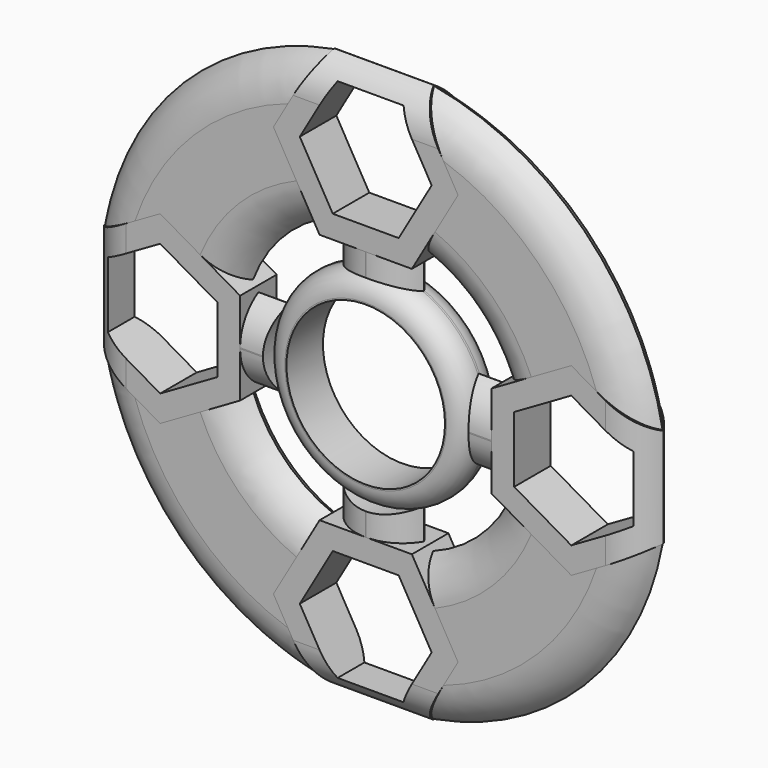
from build123d import *

# Parameters (mm, degrees)
F0_R          = 14.2875
F0_R_2        = 11.0236
F2_DEPTH      = 6.35
F3_T2_ANGLE   = 116.8949304421
F3_T4_ANGLE   = 116.8949304421
F3_2_T2_ANGLE = 116.8949304421
F3_2_T4_ANGLE = 116.8949304421
F3_3_T2_ANGLE = 116.8949304421
F3_3_T4_ANGLE = 116.8949304421
F3_4_T2_ANGLE = 116.8949304421
F3_4_T4_ANGLE = 116.8949304421
F3_5_T1_DEPTH = 44.5816097327
F3_6_T1_DEPTH = 44.5816097327
F3_7_T1_DEPTH = 44.5816097327
F3_8_T1_DEPTH = 44.5816097327
F4_T1_DEPTH   = 36.4465255301
F4_2_T1_DEPTH = 36.4465255301
F4_3_T1_DEPTH = 36.4465255301
F4_4_T1_DEPTH = 36.4465255301
F5_T2_ANGLE   = 147.4481035584
F5_T4_ANGLE   = 147.4481035584
F5_2_T2_ANGLE = 147.4481035584
F5_2_T4_ANGLE = 147.4481035584
F5_3_T2_ANGLE = 147.4481035584
F5_3_T4_ANGLE = 147.4481035584
F5_4_T2_ANGLE = 147.4481035584
F5_4_T4_ANGLE = 147.4481035584
F6_R          = 3.048


# Not quite as in the source:
# - a fillet or chamfer that OpenCascade refuses, or shapes differently, is made with other operations: its cross-section is extruded or revolved along the edge and cut away or added


with BuildPart() as f2:
    # F0 (on Front) → F2 (new body)
    with BuildSketch(Plane.XZ):
        Circle(F0_R)
        Circle(F0_R_2, mode=Mode.SUBTRACT)
    extrude(amount=F2_DEPTH)

    # F6
    f6_edges = [f2.edges().sort_by_distance(p)[0] for p in [
        (-14.2875, 0, 0),
        (-14.2875, -6.35, 0),
    ]]
    fillet(f6_edges, radius=F6_R)


with BuildPart() as f2b:
    # F0 (on Front) → F2, piece 2 (new body)
    with BuildSketch(Plane.XZ):
        Polygon((-6.4158048664, 17.4625), (6.4158048664, 17.4625), (12.8316097327, 28.575), (6.4158048664, 39.6875), (-6.4158048664, 39.6875), (-12.8316097327, 28.575), align=None)
        Polygon((9.1654355234, 28.575), (4.5827177617, 20.6375), (-4.5827177617, 20.6375), (-9.1654355234, 28.575), (-4.5827177617, 36.5125), (4.5827177617, 36.5125), align=None, mode=Mode.SUBTRACT)
    extrude(amount=F2_DEPTH)

    # F3#5: fillet of radius 6.35 on 2 edges, made by hand

    # F3_5_s2 → F3_5_t1 (cut)
    with BuildSketch(Plane.YZ.offset(-22.2908048664)):
        with BuildLine():
            ThreePointArc((0, 39.6875), (-4.4901280605, 37.8276280605), (-6.35, 33.3375))
            Line((-6.35, 33.3375), (-6.35, 39.6875))
            Line((-6.35, 39.6875), (0, 39.6875))
        make_face()
        with BuildLine():
            ThreePointArc((-6.35, 39.6875), (-1.8598719395, 37.8276280605), (0, 33.3375))
            Line((0, 33.3375), (0, 39.6875))
            Line((0, 39.6875), (-6.35, 39.6875))
        make_face()
    extrude(amount=F3_5_T1_DEPTH, mode=Mode.SUBTRACT)


with BuildPart() as f2c:
    # F0 (on Front) → F2, piece 3 (new body)
    with BuildSketch(Plane.XZ):
        Polygon((-17.4625, 6.4158048664), (-28.575, 12.8316097327), (-39.6875, 6.4158048664), (-39.6875, -6.4158048664), (-28.575, -12.8316097327), (-17.4625, -6.4158048664), align=None)
        Polygon((-28.575, 9.1654355234), (-20.6375, 4.5827177617), (-20.6375, -4.5827177617), (-28.575, -9.1654355234), (-36.5125, -4.5827177617), (-36.5125, 4.5827177617), align=None, mode=Mode.SUBTRACT)
    extrude(amount=F2_DEPTH)

    # F3#6: fillet of radius 6.35 on 2 edges, made by hand

    # F3_6_s2 → F3_6_t1 (cut)
    with BuildSketch(Plane.XY.offset(-22.2908048664)):
        with BuildLine():
            ThreePointArc((-39.6875, 0), (-37.8276280605, -4.4901280605), (-33.3375, -6.35))
            Line((-33.3375, -6.35), (-39.6875, -6.35))
            Line((-39.6875, -6.35), (-39.6875, 0))
        make_face()
        with BuildLine():
            ThreePointArc((-39.6875, -6.35), (-37.8276280605, -1.8598719395), (-33.3375, 0))
            Line((-33.3375, 0), (-39.6875, 0))
            Line((-39.6875, 0), (-39.6875, -6.35))
        make_face()
    extrude(amount=F3_6_T1_DEPTH, mode=Mode.SUBTRACT)


with BuildPart() as f2d:
    # F0 (on Front) → F2, piece 4 (new body)
    with BuildSketch(Plane.XZ):
        Polygon((-6.4158048664, -17.4625), (-12.8316097327, -28.575), (-6.4158048664, -39.6875), (6.4158048664, -39.6875), (12.8316097327, -28.575), (6.4158048664, -17.4625), align=None)
        Polygon((-9.1654355234, -28.575), (-4.5827177617, -20.6375), (4.5827177617, -20.6375), (9.1654355234, -28.575), (4.5827177617, -36.5125), (-4.5827177617, -36.5125), align=None, mode=Mode.SUBTRACT)
    extrude(amount=F2_DEPTH)

    # F3#8: fillet of radius 6.35 on 2 edges, made by hand

    # F3_8_s2 → F3_8_t1 (cut)
    with BuildSketch(Plane.YZ.offset(-22.2908048664)):
        with BuildLine():
            ThreePointArc((0, -39.6875), (-4.4901280605, -37.8276280605), (-6.35, -33.3375))
            Line((-6.35, -33.3375), (-6.35, -39.6875))
            Line((-6.35, -39.6875), (0, -39.6875))
        make_face()
        with BuildLine():
            ThreePointArc((-6.35, -39.6875), (-1.8598719395, -37.8276280605), (0, -33.3375))
            Line((0, -33.3375), (0, -39.6875))
            Line((0, -39.6875), (-6.35, -39.6875))
        make_face()
    extrude(amount=F3_8_T1_DEPTH, mode=Mode.SUBTRACT)


with BuildPart() as f2e:
    # F0 (on Front) → F2, piece 5 (new body)
    with BuildSketch(Plane.XZ):
        Polygon((17.4625, -6.4158048664), (28.575, -12.8316097327), (39.6875, -6.4158048664), (39.6875, 6.4158048664), (28.575, 12.8316097327), (17.4625, 6.4158048664), align=None)
        Polygon((28.575, -9.1654355234), (20.6375, -4.5827177617), (20.6375, 4.5827177617), (28.575, 9.1654355234), (36.5125, 4.5827177617), (36.5125, -4.5827177617), align=None, mode=Mode.SUBTRACT)
    extrude(amount=F2_DEPTH)

    # F3#7: fillet of radius 6.35 on 2 edges, made by hand

    # F3_7_s2 → F3_7_t1 (cut)
    with BuildSketch(Plane.XY.offset(-22.2908048664)):
        with BuildLine():
            ThreePointArc((39.6875, 0), (37.8276280605, -4.4901280605), (33.3375, -6.35))
            Line((33.3375, -6.35), (39.6875, -6.35))
            Line((39.6875, -6.35), (39.6875, 0))
        make_face()
        with BuildLine():
            ThreePointArc((39.6875, -6.35), (37.8276280605, -1.8598719395), (33.3375, 0))
            Line((33.3375, 0), (39.6875, 0))
            Line((39.6875, 0), (39.6875, -6.35))
        make_face()
    extrude(amount=F3_7_T1_DEPTH, mode=Mode.SUBTRACT)


with BuildPart() as f2f:
    # F1 (on Front) → F2, piece 6 (new body)
    with BuildSketch(Plane.XZ):
        with BuildLine():
            ThreePointArc((-6.4158048664, 39.6875), (-28.4276292393, 28.4276292393), (-39.6875, 6.4158048664))
            Line((-39.6875, 6.4158048664), (-34.1312501453, 9.6237072156))
            Line((-34.1312501453, 9.6237072156), (-28.575, 12.8316097327))
            Line((-28.575, 12.8316097327), (-23.0187499915, 9.6237072946))
            Line((-23.0187499915, 9.6237072946), (-17.4625, 6.4158048664))
            ThreePointArc((-17.4625, 6.4158048664), (-13.1548747302, 13.1548747302), (-6.4158048664, 17.4625))
            Line((-6.4158048664, 17.4625), (-9.6237073033, 23.0187500066))
            Line((-9.6237073033, 23.0187500066), (-12.8316097327, 28.575))
            Line((-12.8316097327, 28.575), (-9.6237073033, 34.1312499934))
            Line((-9.6237073033, 34.1312499934), (-6.4158048664, 39.6875))
        make_face()
    extrude(amount=F2_DEPTH)

    # F3#4: fillet of radius 6.35 on 2 edges, made by hand

    # F3_4_s1 → F3_4_t2 (revolve, cut)
    with BuildSketch(Plane(origin=(0, 0, 0), x_dir=(0, 1, 0), z_dir=(0.9725835588, 0, -0.2325536951))):
        with BuildLine():
            ThreePointArc((0, 40.2027388163), (-4.4901280605, 38.3428668769), (-6.35, 33.8527388163))
            Line((-6.35, 33.8527388163), (-6.35, 40.2027388163))
            Line((-6.35, 40.2027388163), (0, 40.2027388163))
        make_face()
    revolve(axis=Axis((0, -6.35, 0), (0, -1, 0)), revolution_arc=F3_4_T2_ANGLE, mode=Mode.SUBTRACT)

    # F3_4_s3 → F3_4_t4 (revolve, cut)
    with BuildSketch(Plane(origin=(0, 0, 0), x_dir=(0, 1, 0), z_dir=(0.9725835588, 0, -0.2325536951))):
        with BuildLine():
            ThreePointArc((0, 33.8527388163), (-1.8598719395, 38.3428668769), (-6.35, 40.2027388163))
            Line((-6.35, 40.2027388163), (0, 40.2027388163))
            Line((0, 40.2027388163), (0, 33.8527388163))
        make_face()
    revolve(axis=Axis((0, 0, 0), (0, -1, 0)), revolution_arc=F3_4_T4_ANGLE, mode=Mode.SUBTRACT)

    # F5: fillet of radius 6.35 on 2 edges, made by hand

    # F5_s1 → F5_t2 (revolve, cut)
    with BuildSketch(Plane(origin=(0, 0, 0), x_dir=(0, 1, 0), z_dir=(0.4805916659, 0, -0.8769444969))):
        with BuildLine():
            ThreePointArc((-6.35, -24.9538022547), (-4.4901280605, -20.4636741942), (0, -18.6038022547))
            Line((0, -18.6038022547), (-6.35, -18.6038022547))
            Line((-6.35, -18.6038022547), (-6.35, -24.9538022547))
        make_face()
    revolve(axis=Axis((0, -6.35, 0), (0, 1, 0)), revolution_arc=F5_T2_ANGLE, mode=Mode.SUBTRACT)

    # F5_s3 → F5_t4 (revolve, cut)
    with BuildSketch(Plane(origin=(0, 0, 0), x_dir=(0, 1, 0), z_dir=(0.4805916659, 0, -0.8769444969))):
        with BuildLine():
            ThreePointArc((0, -24.9538022547), (-1.8598719395, -20.4636741942), (-6.35, -18.6038022547))
            Line((-6.35, -18.6038022547), (0, -18.6038022547))
            Line((0, -18.6038022547), (0, -24.9538022547))
        make_face()
    revolve(axis=Axis((0, 0, 0), (0, 1, 0)), revolution_arc=F5_T4_ANGLE, mode=Mode.SUBTRACT)


with BuildPart() as f2g:
    # F1 (on Front) → F2, piece 7 (new body)
    with BuildSketch(Plane.XZ):
        with BuildLine():
            Line((34.1312500085, 9.6237072946), (39.6875, 6.4158048664))
            ThreePointArc((39.6875, 6.4158048664), (28.4276292393, 28.4276292393), (6.4158048664, 39.6875))
            Line((6.4158048664, 39.6875), (9.6237073207, 34.1312499633))
            Line((9.6237073207, 34.1312499633), (12.8316097327, 28.575))
            Line((12.8316097327, 28.575), (9.6237072806, 23.0187499671))
            Line((9.6237072806, 23.0187499671), (6.4158048664, 17.4625))
            ThreePointArc((6.4158048664, 17.4625), (13.1548747302, 13.1548747302), (17.4625, 6.4158048664))
            Line((17.4625, 6.4158048664), (23.0187500159, 9.6237073087))
            Line((23.0187500159, 9.6237073087), (28.575, 12.8316097327))
            Line((28.575, 12.8316097327), (34.1312500085, 9.6237072946))
        make_face()
    extrude(amount=F2_DEPTH)

    # F3: fillet of radius 6.35 on 2 edges, made by hand

    # F3_s1 → F3_t2 (revolve, cut)
    with BuildSketch(Plane(origin=(0, 0, 0), x_dir=(0, 1, 0), z_dir=(-0.2325536951, 0, -0.9725835588))):
        with BuildLine():
            ThreePointArc((0, 40.2027388163), (-4.4901280605, 38.3428668769), (-6.35, 33.8527388163))
            Line((-6.35, 33.8527388163), (-6.35, 40.2027388163))
            Line((-6.35, 40.2027388163), (0, 40.2027388163))
        make_face()
    revolve(axis=Axis((0, -6.35, 0), (0, -1, 0)), revolution_arc=F3_T2_ANGLE, mode=Mode.SUBTRACT)

    # F3_s3 → F3_t4 (revolve, cut)
    with BuildSketch(Plane(origin=(0, 0, 0), x_dir=(0, 1, 0), z_dir=(-0.2325536951, 0, -0.9725835588))):
        with BuildLine():
            ThreePointArc((0, 33.8527388163), (-1.8598719395, 38.3428668769), (-6.35, 40.2027388163))
            Line((-6.35, 40.2027388163), (0, 40.2027388163))
            Line((0, 40.2027388163), (0, 33.8527388163))
        make_face()
    revolve(axis=Axis((0, 0, 0), (0, -1, 0)), revolution_arc=F3_T4_ANGLE, mode=Mode.SUBTRACT)

    # F5#4: fillet of radius 6.35 on 2 edges, made by hand

    # F5_4_s1 → F5_4_t2 (revolve, cut)
    with BuildSketch(Plane(origin=(0, 0, 0), x_dir=(0, 1, 0), z_dir=(-0.8769444969, 0, -0.4805916659))):
        with BuildLine():
            ThreePointArc((-6.35, -24.9538022547), (-4.4901280605, -20.4636741942), (0, -18.6038022547))
            Line((0, -18.6038022547), (-6.35, -18.6038022547))
            Line((-6.35, -18.6038022547), (-6.35, -24.9538022547))
        make_face()
    revolve(axis=Axis((0, -6.35, 0), (0, 1, 0)), revolution_arc=F5_4_T2_ANGLE, mode=Mode.SUBTRACT)

    # F5_4_s3 → F5_4_t4 (revolve, cut)
    with BuildSketch(Plane(origin=(0, 0, 0), x_dir=(0, 1, 0), z_dir=(-0.8769444969, 0, -0.4805916659))):
        with BuildLine():
            ThreePointArc((0, -24.9538022547), (-1.8598719395, -20.4636741942), (-6.35, -18.6038022547))
            Line((-6.35, -18.6038022547), (0, -18.6038022547))
            Line((0, -18.6038022547), (0, -24.9538022547))
        make_face()
    revolve(axis=Axis((0, 0, 0), (0, 1, 0)), revolution_arc=F5_4_T4_ANGLE, mode=Mode.SUBTRACT)


with BuildPart() as f2h:
    # F1 (on Front) → F2, piece 8 (new body)
    with BuildSketch(Plane.XZ):
        with BuildLine():
            Line((9.6237072946, -23.0187499915), (12.8316097327, -28.575))
            Line((12.8316097327, -28.575), (9.6237072946, -34.1312500085))
            Line((9.6237072946, -34.1312500085), (6.4158048664, -39.6875))
            ThreePointArc((6.4158048664, -39.6875), (28.4276292393, -28.4276292393), (39.6875, -6.4158048664))
            Line((39.6875, -6.4158048664), (34.1312500668, -9.623707261))
            Line((34.1312500668, -9.623707261), (28.575, -12.8316097327))
            Line((28.575, -12.8316097327), (23.0187499915, -9.6237072946))
            Line((23.0187499915, -9.6237072946), (17.4625, -6.4158048664))
            ThreePointArc((17.4625, -6.4158048664), (13.1548747302, -13.1548747302), (6.4158048664, -17.4625))
            Line((6.4158048664, -17.4625), (9.6237072946, -23.0187499915))
        make_face()
    extrude(amount=F2_DEPTH)

    # F3#2: fillet of radius 6.35 on 2 edges, made by hand

    # F3_2_s1 → F3_2_t2 (revolve, cut)
    with BuildSketch(Plane(origin=(0, 0, 0), x_dir=(0, 1, 0), z_dir=(-0.9725835588, 0, 0.2325536951))):
        with BuildLine():
            ThreePointArc((-6.35, 33.8527388163), (-4.4901280605, 38.3428668769), (0, 40.2027388163))
            Line((0, 40.2027388163), (-6.35, 40.2027388163))
            Line((-6.35, 40.2027388163), (-6.35, 33.8527388163))
        make_face()
    revolve(axis=Axis((0, -6.35, 0), (0, -1, 0)), revolution_arc=F3_2_T2_ANGLE, mode=Mode.SUBTRACT)

    # F3_2_s3 → F3_2_t4 (revolve, cut)
    with BuildSketch(Plane(origin=(0, 0, 0), x_dir=(0, 1, 0), z_dir=(-0.9725835588, 0, 0.2325536951))):
        with BuildLine():
            ThreePointArc((0, 33.8527388163), (-1.8598719395, 38.3428668769), (-6.35, 40.2027388163))
            Line((-6.35, 40.2027388163), (0, 40.2027388163))
            Line((0, 40.2027388163), (0, 33.8527388163))
        make_face()
    revolve(axis=Axis((0, 0, 0), (0, -1, 0)), revolution_arc=F3_2_T4_ANGLE, mode=Mode.SUBTRACT)

    # F5#3: fillet of radius 6.35 on 2 edges, made by hand

    # F5_3_s1 → F5_3_t2 (revolve, cut)
    with BuildSketch(Plane(origin=(0, 0, 0), x_dir=(0, 1, 0), z_dir=(-0.4805916659, 0, 0.8769444969))):
        with BuildLine():
            ThreePointArc((-6.35, -24.9538022547), (-4.4901280605, -20.4636741942), (0, -18.6038022547))
            Line((0, -18.6038022547), (-6.35, -18.6038022547))
            Line((-6.35, -18.6038022547), (-6.35, -24.9538022547))
        make_face()
    revolve(axis=Axis((0, -6.35, 0), (0, 1, 0)), revolution_arc=F5_3_T2_ANGLE, mode=Mode.SUBTRACT)

    # F5_3_s3 → F5_3_t4 (revolve, cut)
    with BuildSketch(Plane(origin=(0, 0, 0), x_dir=(0, 1, 0), z_dir=(-0.4805916659, 0, 0.8769444969))):
        with BuildLine():
            ThreePointArc((0, -24.9538022547), (-1.8598719395, -20.4636741942), (-6.35, -18.6038022547))
            Line((-6.35, -18.6038022547), (0, -18.6038022547))
            Line((0, -18.6038022547), (0, -24.9538022547))
        make_face()
    revolve(axis=Axis((0, 0, 0), (0, 1, 0)), revolution_arc=F5_3_T4_ANGLE, mode=Mode.SUBTRACT)


with BuildPart() as f2i:
    # F1 (on Front) → F2, piece 9 (new body)
    with BuildSketch(Plane.XZ):
        with BuildLine():
            ThreePointArc((-39.6875, -6.4158048664), (-28.4276292393, -28.4276292393), (-6.4158048664, -39.6875))
            Line((-6.4158048664, -39.6875), (-9.6237073033, -34.1312499934))
            Line((-9.6237073033, -34.1312499934), (-12.8316097327, -28.575))
            Line((-12.8316097327, -28.575), (-9.6237072946, -23.0187499915))
            Line((-9.6237072946, -23.0187499915), (-6.4158048664, -17.4625))
            ThreePointArc((-6.4158048664, -17.4625), (-13.1548747302, -13.1548747302), (-17.4625, -6.4158048664))
            Line((-17.4625, -6.4158048664), (-23.0187500065, -9.6237073033))
            Line((-23.0187500065, -9.6237073033), (-28.575, -12.8316097327))
            Line((-28.575, -12.8316097327), (-34.1312500329, -9.6237072806))
            Line((-34.1312500329, -9.6237072806), (-39.6875, -6.4158048664))
        make_face()
    extrude(amount=F2_DEPTH)

    # F3#3: fillet of radius 6.35 on 2 edges, made by hand

    # F3_3_s1 → F3_3_t2 (revolve, cut)
    with BuildSketch(Plane(origin=(0, 0, 0), x_dir=(0, 1, 0), z_dir=(0.2325536951, 0, 0.9725835588))):
        with BuildLine():
            ThreePointArc((0, 40.2027388163), (-4.4901280605, 38.3428668769), (-6.35, 33.8527388163))
            Line((-6.35, 33.8527388163), (-6.35, 40.2027388163))
            Line((-6.35, 40.2027388163), (0, 40.2027388163))
        make_face()
    revolve(axis=Axis((0, -6.35, 0), (0, -1, 0)), revolution_arc=F3_3_T2_ANGLE, mode=Mode.SUBTRACT)

    # F3_3_s3 → F3_3_t4 (revolve, cut)
    with BuildSketch(Plane(origin=(0, 0, 0), x_dir=(0, 1, 0), z_dir=(0.2325536951, 0, 0.9725835588))):
        with BuildLine():
            ThreePointArc((-6.35, 40.2027388163), (-1.8598719395, 38.3428668769), (0, 33.8527388163))
            Line((0, 33.8527388163), (0, 40.2027388163))
            Line((0, 40.2027388163), (-6.35, 40.2027388163))
        make_face()
    revolve(axis=Axis((0, 0, 0), (0, -1, 0)), revolution_arc=F3_3_T4_ANGLE, mode=Mode.SUBTRACT)

    # F5#2: fillet of radius 6.35 on 2 edges, made by hand

    # F5_2_s1 → F5_2_t2 (revolve, cut)
    with BuildSketch(Plane(origin=(0, 0, 0), x_dir=(0, 1, 0), z_dir=(0.8769444969, 0, 0.4805916659))):
        with BuildLine():
            ThreePointArc((0, -18.6038022547), (-4.4901280605, -20.4636741942), (-6.35, -24.9538022547))
            Line((-6.35, -24.9538022547), (-6.35, -18.6038022547))
            Line((-6.35, -18.6038022547), (0, -18.6038022547))
        make_face()
    revolve(axis=Axis((0, -6.35, 0), (0, 1, 0)), revolution_arc=F5_2_T2_ANGLE, mode=Mode.SUBTRACT)

    # F5_2_s3 → F5_2_t4 (revolve, cut)
    with BuildSketch(Plane(origin=(0, 0, 0), x_dir=(0, 1, 0), z_dir=(0.8769444969, 0, 0.4805916659))):
        with BuildLine():
            ThreePointArc((0, -24.9538022547), (-1.8598719395, -20.4636741942), (-6.35, -18.6038022547))
            Line((-6.35, -18.6038022547), (0, -18.6038022547))
            Line((0, -18.6038022547), (0, -24.9538022547))
        make_face()
    revolve(axis=Axis((0, 0, 0), (0, 1, 0)), revolution_arc=F5_2_T4_ANGLE, mode=Mode.SUBTRACT)


with BuildPart() as f2j:
    # F1 (on Front) → F2, piece 10 (new body)
    with BuildSketch(Plane.XZ):
        with BuildLine():
            Line((0, -17.4625), (6.4158048664, -17.4625))
            Line((6.4158048664, -17.4625), (6.4158048664, -12.7659744699))
            ThreePointArc((6.4158048664, -12.7659744699), (0, -14.2875), (-6.4158048664, -12.7659744699))
            Line((-6.4158048664, -12.7659744699), (-6.4158048664, -17.4625))
            Line((-6.4158048664, -17.4625), (0, -17.4625))
        make_face()
    extrude(amount=F2_DEPTH)

    # F4: fillet of radius 6.35 on 4 edges, made by hand

    # F4_s2 → F4_t1 (cut)
    with BuildSketch(Plane.XY.offset(-33.3375)):
        with BuildLine():
            ThreePointArc((6.4158048664, 0), (4.5559329269, -4.4901280605), (0.0658048664, -6.35))
            Line((0.0658048664, -6.35), (6.4158048664, -6.35))
            Line((6.4158048664, -6.35), (6.4158048664, 0))
        make_face()
        with BuildLine():
            ThreePointArc((-0.0658048664, -6.35), (-4.5559329269, -4.4901280605), (-6.4158048664, 0))
            Line((-6.4158048664, 0), (-6.4158048664, -6.35))
            Line((-6.4158048664, -6.35), (-0.0658048664, -6.35))
        make_face()
        with BuildLine():
            ThreePointArc((0.0658048664, 0), (4.5559329269, -1.8598719395), (6.4158048664, -6.35))
            Line((6.4158048664, -6.35), (6.4158048664, 0))
            Line((6.4158048664, 0), (0.0658048664, 0))
        make_face()
        with BuildLine():
            ThreePointArc((-0.0658048664, 0), (-4.5559329269, -1.8598719395), (-6.4158048664, -6.35))
            Line((-6.4158048664, -6.35), (-6.4158048664, 0))
            Line((-6.4158048664, 0), (-0.0658048664, 0))
        make_face()
    extrude(amount=F4_T1_DEPTH, mode=Mode.SUBTRACT)


with BuildPart() as f2k:
    # F1 (on Front) → F2, piece 11 (new body)
    with BuildSketch(Plane.XZ):
        with BuildLine():
            Line((12.7659744699, -6.4158048664), (17.4625, -6.4158048664))
            Line((17.4625, -6.4158048664), (17.4625, 0))
            Line((17.4625, 0), (17.4625, 6.4158048664))
            Line((17.4625, 6.4158048664), (12.7659744699, 6.4158048664))
            ThreePointArc((12.7659744699, 6.4158048664), (13.9019156322, 3.2968770079), (14.2875, 0))
            ThreePointArc((14.2875, 0), (13.9019156322, -3.2968770079), (12.7659744699, -6.4158048664))
        make_face()
    extrude(amount=F2_DEPTH)

    # F4#4: fillet of radius 6.35 on 4 edges, made by hand

    # F4_4_s2 → F4_4_t1 (cut)
    with BuildSketch(Plane.YZ.offset(-3.1090255301)):
        with BuildLine():
            ThreePointArc((-6.35, 0.0658048664), (-4.4901280605, 4.5559329269), (0, 6.4158048664))
            Line((0, 6.4158048664), (-6.35, 6.4158048664))
            Line((-6.35, 6.4158048664), (-6.35, 0.0658048664))
        make_face()
        with BuildLine():
            ThreePointArc((-6.35, -0.0658048664), (-4.4901280605, -4.5559329269), (0, -6.4158048664))
            Line((0, -6.4158048664), (-6.35, -6.4158048664))
            Line((-6.35, -6.4158048664), (-6.35, -0.0658048664))
        make_face()
        with BuildLine():
            ThreePointArc((-6.35, 6.4158048664), (-1.8598719395, 4.5559329269), (0, 0.0658048664))
            Line((0, 0.0658048664), (0, 6.4158048664))
            Line((0, 6.4158048664), (-6.35, 6.4158048664))
        make_face()
        with BuildLine():
            ThreePointArc((0, -0.0658048664), (-1.8598719395, -4.5559329269), (-6.35, -6.4158048664))
            Line((-6.35, -6.4158048664), (0, -6.4158048664))
            Line((0, -6.4158048664), (0, -0.0658048664))
        make_face()
    extrude(amount=F4_4_T1_DEPTH, mode=Mode.SUBTRACT)


with BuildPart() as f2l:
    # F1 (on Front) → F2, piece 12 (new body)
    with BuildSketch(Plane.XZ):
        with BuildLine():
            Line((6.4158048664, 12.7659744699), (6.4158048664, 17.4625))
            Line((6.4158048664, 17.4625), (0, 17.4625))
            Line((0, 17.4625), (-6.4158048664, 17.4625))
            Line((-6.4158048664, 17.4625), (-6.4158048664, 12.7659744699))
            ThreePointArc((-6.4158048664, 12.7659744699), (0, 14.2875), (6.4158048664, 12.7659744699))
        make_face()
    extrude(amount=F2_DEPTH)

    # F4#3: fillet of radius 6.35 on 4 edges, made by hand

    # F4_3_s2 → F4_3_t1 (cut)
    with BuildSketch(Plane.XY.offset(-3.1090255301)):
        with BuildLine():
            ThreePointArc((-0.0658048664, -6.35), (-4.5559329269, -4.4901280605), (-6.4158048664, 0))
            Line((-6.4158048664, 0), (-6.4158048664, -6.35))
            Line((-6.4158048664, -6.35), (-0.0658048664, -6.35))
        make_face()
        with BuildLine():
            ThreePointArc((6.4158048664, 0), (4.5559329269, -4.4901280605), (0.0658048664, -6.35))
            Line((0.0658048664, -6.35), (6.4158048664, -6.35))
            Line((6.4158048664, -6.35), (6.4158048664, 0))
        make_face()
        with BuildLine():
            ThreePointArc((-6.4158048664, -6.35), (-4.5559329269, -1.8598719395), (-0.0658048664, 0))
            Line((-0.0658048664, 0), (-6.4158048664, 0))
            Line((-6.4158048664, 0), (-6.4158048664, -6.35))
        make_face()
        with BuildLine():
            ThreePointArc((6.4158048664, -6.35), (4.5559329269, -1.8598719395), (0.0658048664, 0))
            Line((0.0658048664, 0), (6.4158048664, 0))
            Line((6.4158048664, 0), (6.4158048664, -6.35))
        make_face()
    extrude(amount=F4_3_T1_DEPTH, mode=Mode.SUBTRACT)


with BuildPart() as f2m:
    # F1 (on Front) → F2, piece 13 (new body)
    with BuildSketch(Plane.XZ):
        with BuildLine():
            Line((-17.4625, 0), (-17.4625, -6.4158048664))
            Line((-17.4625, -6.4158048664), (-12.7659744699, -6.4158048664))
            ThreePointArc((-12.7659744699, -6.4158048664), (-14.2875, 0), (-12.7659744699, 6.4158048664))
            Line((-12.7659744699, 6.4158048664), (-17.4625, 6.4158048664))
            Line((-17.4625, 6.4158048664), (-17.4625, 0))
        make_face()
    extrude(amount=F2_DEPTH)

    # F4#2: fillet of radius 6.35 on 4 edges, made by hand

    # F4_2_s2 → F4_2_t1 (cut)
    with BuildSketch(Plane.YZ.offset(-33.3375)):
        with BuildLine():
            ThreePointArc((0, -6.4158048664), (-4.4901280605, -4.5559329269), (-6.35, -0.0658048664))
            Line((-6.35, -0.0658048664), (-6.35, -6.4158048664))
            Line((-6.35, -6.4158048664), (0, -6.4158048664))
        make_face()
        with BuildLine():
            ThreePointArc((-6.35, 0.0658048664), (-4.4901280605, 4.5559329269), (0, 6.4158048664))
            Line((0, 6.4158048664), (-6.35, 6.4158048664))
            Line((-6.35, 6.4158048664), (-6.35, 0.0658048664))
        make_face()
        with BuildLine():
            ThreePointArc((0, -0.0658048664), (-1.8598719395, -4.5559329269), (-6.35, -6.4158048664))
            Line((-6.35, -6.4158048664), (0, -6.4158048664))
            Line((0, -6.4158048664), (0, -0.0658048664))
        make_face()
        with BuildLine():
            ThreePointArc((0, 0.0658048664), (-1.8598719395, 4.5559329269), (-6.35, 6.4158048664))
            Line((-6.35, 6.4158048664), (0, 6.4158048664))
            Line((0, 6.4158048664), (0, 0.0658048664))
        make_face()
    extrude(amount=F4_2_T1_DEPTH, mode=Mode.SUBTRACT)


solid = Compound([f2.part, f2b.part, f2c.part, f2d.part, f2e.part, f2f.part, f2g.part, f2h.part, f2i.part, f2j.part, f2k.part, f2l.part, f2m.part])
